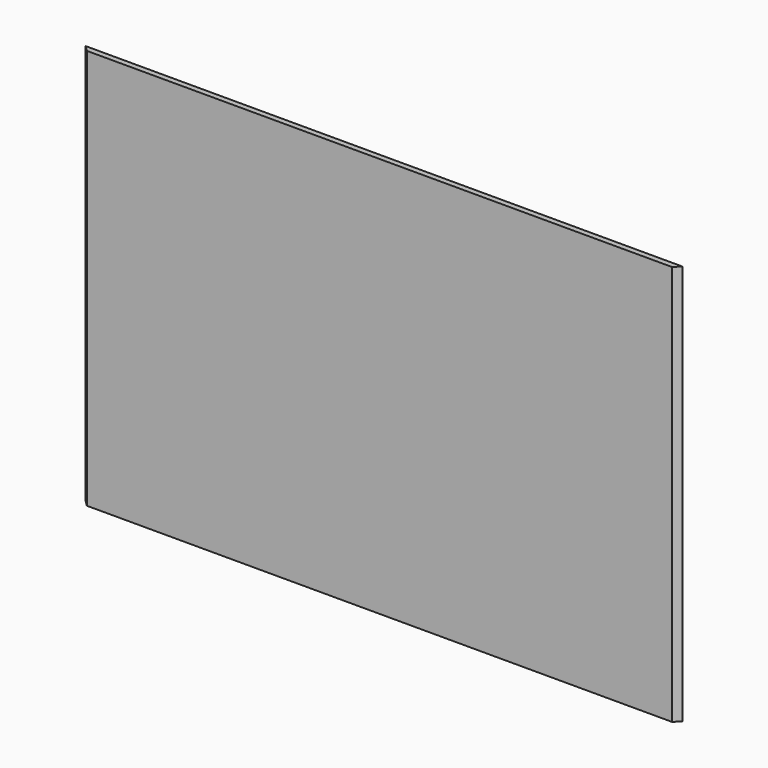
from build123d import *

# Parameters (mm, degrees)
F0_W     = 1460
F0_H     = 980
F1_DEPTH = 14
F2_SIZE  = 13.99999


# Not quite as in the source:
# - a fillet or chamfer is up to 0.001 mm smaller than in the source, because OpenCascade refuses the exact size


with BuildPart() as f1:
    # F0 (on Front) → F1 (new body)
    with BuildSketch(Plane.XZ):
        Rectangle(F0_W, F0_H)
    extrude(amount=F1_DEPTH)

    # F2 (size 14 in the source; OpenCascade refuses exactly that, so slightly less here)
    f2_edges = [f1.edges().sort_by_distance(p)[0] for p in [
        (-730, -14, 0),
        (730, -14, 0),
    ]]
    chamfer(f2_edges, length=F2_SIZE)


solid = f1.part
